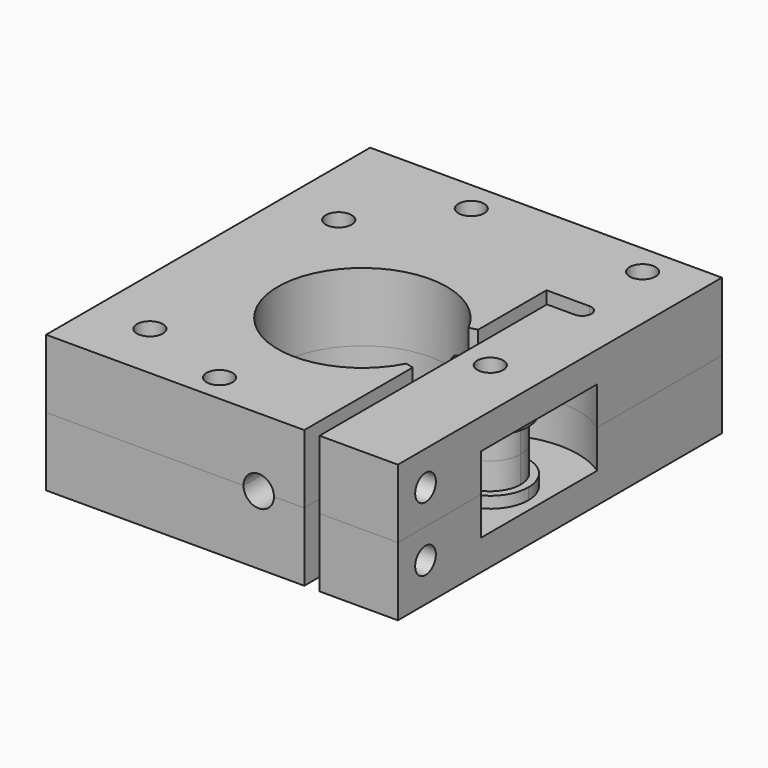
from build123d import *

# Parameters (mm, degrees)
F0_R           = 1.7
F0_R_2         = 1.35
F1_DEPTH       = 9
F2_R           = 11.1
F2_R_2         = 1.7
F3_DEPTH       = 9.001
F5_DEPTH       = 5
F6_DEPTH       = 3.5
F11_DEPTH      = 9
F13_DEPTH      = 9.001
F14_DEPTH      = 5
F15_DEPTH      = 3.5
F18_R          = 1.4
F19_DEPTH      = 20
F18_R_2        = 1.7
F20_DEPTH      = 11
F21_DEPTH      = 20
F22_DEPTH      = 11
F4_R           = 1.4
F23_DEPTH      = 9.0010001
F4_R_2         = 1.7
F24_DEPTH      = 9.0010001
F25_T1_DEPTH   = 25.9070070941
F25_2_T1_DEPTH = 25.9070070941


# Not quite as in the source:
# - a fillet or chamfer that OpenCascade refuses, or shapes differently, is made with other operations: its cross-section is extruded or revolved along the edge and cut away or added


with BuildPart() as f1:
    # F0 (on Top) → F1 (new body)
    with BuildSketch(Plane.XY):
        with BuildLine():
            Line((21.7747555523, 35.8522933333), (-24.4267012457, 35.8522933333))
            Line((-24.4267012457, 35.8522933333), (-24.4267012457, -17.3452516382))
            Line((-24.4267012457, -17.3452516382), (9.4824641046, -17.3452516382))
            Line((9.4824641046, -17.3452516382), (9.4824641046, 22.4300473309))
            Line((9.4824641046, 22.4300473309), (15.1353199035, 22.4300473309))
            ThreePointArc((15.1353199035, 22.4300473309), (16.352897448, 21.2124697864), (15.1353199035, 19.9948922419))
            Line((15.1353199035, 19.9948922419), (11.4824641046, 19.9948922419))
            Line((11.4824641046, 19.9948922419), (11.4824641046, -17.3452516382))
            Line((11.4824641046, -17.3452516382), (21.7747555523, -17.3452516382))
            Line((21.7747555523, -17.3452516382), (21.7747555523, 35.8522933333))
        make_face()
        with Locations((-4.5850900933, -13.6724999174)):
            Circle(F0_R, mode=Mode.SUBTRACT)
        with Locations((-7.8875971958, 31.7803174257)):
            Circle(F0_R, mode=Mode.SUBTRACT)
        with Locations((14.6124028042, 31.7803174257)):
            Circle(F0_R, mode=Mode.SUBTRACT)
        with Locations((-7.8875971958, 31.7803174257)):
            Circle(F0_R)
        with Locations((-7.8875971958, 31.7803174257)):
            Circle(F0_R_2, mode=Mode.SUBTRACT)
        with Locations((14.6124028042, 31.7803174257)):
            Circle(F0_R)
        with Locations((14.6124028042, 31.7803174257)):
            Circle(F0_R_2, mode=Mode.SUBTRACT)
        with Locations((-4.5850900933, -13.6724999174)):
            Circle(F0_R)
        with Locations((-4.5850900933, -13.6724999174)):
            Circle(F0_R_2, mode=Mode.SUBTRACT)
    extrude(amount=F1_DEPTH)

    # F2 (on face) → F3 (cut, through all)
    with BuildSketch(Plane.XY.offset(9)):
        with Locations((-1.4267012457, 5.8241346851)):
            Circle(F2_R)
        with Locations((-16.9267012457, 21.3241346851)):
            Circle(F2_R_2)
        with Locations((-16.9267012457, -9.6758653149)):
            Circle(F2_R_2)
    extrude(amount=-F3_DEPTH, mode=Mode.SUBTRACT)

    # F4 (on face) → F5 (cut)
    with BuildSketch(Plane.XY.offset(9)):
        with BuildLine():
            Line((11.4824641046, 8.9644222084), (11.4824641046, 16.6459370178))
            ThreePointArc((11.4824641046, 16.6459370178), (10.4596854864, 16.2215576665), (9.4824641046, 15.700777188))
            Line((9.4824641046, 15.700777188), (9.4824641046, 7.873552007))
            ThreePointArc((9.4824641046, 7.873552007), (8.4835434412, 10.8238397011), (6.7042511353, 13.380430959))
            ThreePointArc((6.7042511353, 13.380430959), (3.8732987543, 5.8241346851), (6.7042511353, -1.7321615888))
            ThreePointArc((6.7042511353, -1.7321615888), (8.4835434412, 0.8244296691), (9.4824641046, 3.7747173632))
            Line((9.4824641046, 3.7747173632), (9.4824641046, -4.0525078178))
            ThreePointArc((9.4824641046, -4.0525078178), (10.4596854864, -4.5732882963), (11.4824641046, -4.9976676476))
            Line((11.4824641046, -4.9976676476), (11.4824641046, 2.6838471618))
            ThreePointArc((11.4824641046, 2.6838471618), (10.3732987543, 5.8241346851), (11.4824641046, 8.9644222084))
        make_face()
        with BuildLine():
            Line((21.7747555523, -3.7294693921), (21.7747555523, 15.3777387623))
            ThreePointArc((21.7747555523, 15.3777387623), (16.7796726722, 17.2378156165), (11.4824641046, 16.6459370178))
            Line((11.4824641046, 16.6459370178), (11.4824641046, 8.9644222084))
            ThreePointArc((11.4824641046, 8.9644222084), (17.0385054609, 10.5386958125), (20.3732987543, 5.8241346851))
            ThreePointArc((20.3732987543, 5.8241346851), (17.0385054609, 1.1095735577), (11.4824641046, 2.6838471618))
            Line((11.4824641046, 2.6838471618), (11.4824641046, -4.9976676476))
            ThreePointArc((11.4824641046, -4.9976676476), (16.7796726722, -5.5895462463), (21.7747555523, -3.7294693921))
        make_face()
    extrude(amount=-F5_DEPTH, mode=Mode.SUBTRACT)

    # F4 (on face) → F6 (cut)
    with BuildSketch(Plane.XY.offset(9)):
        with BuildLine():
            Line((11.4824641046, 6.7522541434), (11.4824641046, 8.9644222084))
            ThreePointArc((11.4824641046, 8.9644222084), (10.3732987543, 5.8241346851), (11.4824641046, 2.6838471618))
            Line((11.4824641046, 2.6838471618), (11.4824641046, 4.8960152268))
            ThreePointArc((11.4824641046, 4.8960152268), (11.3732987543, 5.8241346851), (11.4824641046, 6.7522541434))
        make_face()
        with BuildLine():
            ThreePointArc((20.3732987543, 5.8241346851), (17.0385054609, 10.5386958125), (11.4824641046, 8.9644222084))
            Line((11.4824641046, 8.9644222084), (11.4824641046, 6.7522541434))
            ThreePointArc((11.4824641046, 6.7522541434), (15.8405574628, 9.7967496047), (19.3732987543, 5.8241346851))
            ThreePointArc((19.3732987543, 5.8241346851), (15.8405574628, 1.8515197655), (11.4824641046, 4.8960152268))
            Line((11.4824641046, 4.8960152268), (11.4824641046, 2.6838471618))
            ThreePointArc((11.4824641046, 2.6838471618), (17.0385054609, 1.1095735577), (20.3732987543, 5.8241346851))
        make_face()
    extrude(amount=-F6_DEPTH, mode=Mode.SUBTRACT)


with BuildPart() as f8:
    # F7 (on face) → F8 (revolve)
    with BuildSketch(Plane.XY.offset(9)):
        Polygon((1.5, 13.6120927054), (3.5, 13.6120927054), (3.5, 36.5408211946), (-2.6, 36.5408211946), (-2.6, 32.3408211946), (-4.7, 32.3408211946), (-4.7, 27.8408211946), (1.5, 27.8408211946), align=None)
    revolve(axis=Axis((3.5, 25.07645695, 9), (0, 1, 0)))


with BuildPart() as f8b:
    # F7 (on face) → F8, piece 2 (revolve)
    with BuildSketch(Plane.XY.offset(9)):
        Polygon((3.5, -24.8925518245), (3.5, -1.9638233352), (1.9, -1.9638233352), (1.9, -2.2529622074), (1.5, -2.2529622074), (1.5, -6.4595437571), (1.5, -11.6595437571), (1.5, -24.8925518245), align=None)
    revolve(axis=Axis((3.5, 25.07645695, 9), (0, 1, 0)))


with BuildPart() as f1_1:
    add(f1.part)

    # F9: cut F8
    add(f8.part, mode=Mode.SUBTRACT)

    # F10: cut F8b
    add(f8b.part, mode=Mode.SUBTRACT)

    # F18 (on face) → F21 (cut)
    with BuildSketch(Plane.YZ.offset(21.7747555523)):
        with Locations((-12.805685401, 5.0852382556)):
            Circle(F18_R)
    extrude(amount=-F21_DEPTH, mode=Mode.SUBTRACT)

    # F18 (on face) → F22 (cut)
    with BuildSketch(Plane.YZ.offset(21.7747555523)):
        with Locations((-12.805685401, 5.0852382556)):
            Circle(F18_R_2)
        with Locations((-12.805685401, 5.0852382556)):
            Circle(F18_R, mode=Mode.SUBTRACT)
    extrude(amount=-F22_DEPTH, mode=Mode.SUBTRACT)

    # F4 (on face) → F23 (cut, through all)
    with BuildSketch(Plane.XY.offset(9)):
        with Locations((15.3732987543, 5.8241346851)):
            Circle(F4_R)
    extrude(amount=-F23_DEPTH, mode=Mode.SUBTRACT)

    # F25: chamfer of 6 on 2 edges, made by hand

    # F25_s2 → F25_t1 (cut)
    with BuildSketch(Plane.XY.offset(-8.453503547)):
        with BuildLine():
            Line((8.1945876053, 10.8760673026), (9.7156342702, 11.2469045278))
            Line((9.7156342702, 11.2469045278), (9.8356342702, 11.2469045278))
            ThreePointArc((9.8356342702, 11.2469045278), (9.6024641046, 9.5602282674), (9.6024641046, 7.873552007))
            Line((9.6024641046, 7.873552007), (9.3645271819, 7.8513961441))
            ThreePointArc((9.3645271819, 7.8513961441), (8.9500807638, 9.4133957688), (8.0880529132, 10.8208372439))
            Line((8.0880529132, 10.8208372439), (8.1945876053, 10.8760673026))
        make_face()
        with BuildLine():
            Line((9.7156342702, 0.4013648424), (8.1945876053, 0.7722020676))
            Line((8.1945876053, 0.7722020676), (8.0880529132, 0.8274321263))
            ThreePointArc((8.0880529132, 0.8274321263), (8.9500807638, 2.2348736014), (9.3645271819, 3.7968732261))
            Line((9.3645271819, 3.7968732261), (9.6024641046, 3.7747173632))
            ThreePointArc((9.6024641046, 3.7747173632), (9.6024641046, 2.0880411028), (9.8356342702, 0.4013648424))
            Line((9.8356342702, 0.4013648424), (9.7156342702, 0.4013648424))
        make_face()
    extrude(amount=F25_T1_DEPTH, mode=Mode.SUBTRACT)


with BuildPart() as f11:
    # F0 (on Top) → F11 (new body)
    with BuildSketch(Plane.XY):
        with BuildLine():
            Line((21.7747555523, 35.8522933333), (-24.4267012457, 35.8522933333))
            Line((-24.4267012457, 35.8522933333), (-24.4267012457, -17.3452516382))
            Line((-24.4267012457, -17.3452516382), (9.4824641046, -17.3452516382))
            Line((9.4824641046, -17.3452516382), (9.4824641046, 22.4300473309))
            Line((9.4824641046, 22.4300473309), (15.1353199035, 22.4300473309))
            ThreePointArc((15.1353199035, 22.4300473309), (16.352897448, 21.2124697864), (15.1353199035, 19.9948922419))
            Line((15.1353199035, 19.9948922419), (11.4824641046, 19.9948922419))
            Line((11.4824641046, 19.9948922419), (11.4824641046, -17.3452516382))
            Line((11.4824641046, -17.3452516382), (21.7747555523, -17.3452516382))
            Line((21.7747555523, -17.3452516382), (21.7747555523, 35.8522933333))
        make_face()
        with Locations((-4.5850900933, -13.6724999174)):
            Circle(F0_R, mode=Mode.SUBTRACT)
        with Locations((-7.8875971958, 31.7803174257)):
            Circle(F0_R, mode=Mode.SUBTRACT)
        with Locations((14.6124028042, 31.7803174257)):
            Circle(F0_R, mode=Mode.SUBTRACT)
    extrude(amount=-F11_DEPTH)


with BuildPart() as f11_1:
    # F12: moved
    add(f11.part.moved(Location((0, 0, 18))))


with BuildPart() as f13_tool:
    # F2 (on face) → F13 (new body, through all)
    with BuildSketch(Plane.XY.offset(9)):
        with Locations((-1.4267012457, 5.8241346851)):
            Circle(F2_R)
        with Locations((-16.9267012457, 21.3241346851)):
            Circle(F2_R_2)
        with Locations((-16.9267012457, -9.6758653149)):
            Circle(F2_R_2)
    extrude(amount=F13_DEPTH)


with BuildPart() as f8_1:
    add(f8.part)

    # F13: cut by f13_tool
    add(f13_tool.part, mode=Mode.SUBTRACT)


with BuildPart() as f8b_1:
    add(f8b.part)

    # F13: cut by f13_tool
    add(f13_tool.part, mode=Mode.SUBTRACT)


with BuildPart() as f11_2:
    add(f11_1.part)

    # F13: cut by f13_tool
    add(f13_tool.part, mode=Mode.SUBTRACT)

    # F4 (on face) → F14 (cut)
    with BuildSketch(Plane.XY.offset(9)):
        with BuildLine():
            Line((21.7747555523, -3.7294693921), (21.7747555523, 15.3777387623))
            ThreePointArc((21.7747555523, 15.3777387623), (16.7796726722, 17.2378156165), (11.4824641046, 16.6459370178))
            Line((11.4824641046, 16.6459370178), (11.4824641046, 8.9644222084))
            ThreePointArc((11.4824641046, 8.9644222084), (17.0385054609, 10.5386958125), (20.3732987543, 5.8241346851))
            ThreePointArc((20.3732987543, 5.8241346851), (17.0385054609, 1.1095735577), (11.4824641046, 2.6838471618))
            Line((11.4824641046, 2.6838471618), (11.4824641046, -4.9976676476))
            ThreePointArc((11.4824641046, -4.9976676476), (16.7796726722, -5.5895462463), (21.7747555523, -3.7294693921))
        make_face()
    extrude(amount=F14_DEPTH, mode=Mode.SUBTRACT)

    # F4 (on face) → F15 (cut)
    with BuildSketch(Plane.XY.offset(9)):
        with BuildLine():
            Line((11.4824641046, 6.7522541434), (11.4824641046, 8.9644222084))
            ThreePointArc((11.4824641046, 8.9644222084), (10.3732987543, 5.8241346851), (11.4824641046, 2.6838471618))
            Line((11.4824641046, 2.6838471618), (11.4824641046, 4.8960152268))
            ThreePointArc((11.4824641046, 4.8960152268), (11.3732987543, 5.8241346851), (11.4824641046, 6.7522541434))
        make_face()
        with BuildLine():
            ThreePointArc((20.3732987543, 5.8241346851), (17.0385054609, 10.5386958125), (11.4824641046, 8.9644222084))
            Line((11.4824641046, 8.9644222084), (11.4824641046, 6.7522541434))
            ThreePointArc((11.4824641046, 6.7522541434), (15.8405574628, 9.7967496047), (19.3732987543, 5.8241346851))
            ThreePointArc((19.3732987543, 5.8241346851), (15.8405574628, 1.8515197655), (11.4824641046, 4.8960152268))
            Line((11.4824641046, 4.8960152268), (11.4824641046, 2.6838471618))
            ThreePointArc((11.4824641046, 2.6838471618), (17.0385054609, 1.1095735577), (20.3732987543, 5.8241346851))
        make_face()
    extrude(amount=F15_DEPTH, mode=Mode.SUBTRACT)

    # F16: cut F8
    add(f8_1.part, mode=Mode.SUBTRACT)

    # F17: cut F8b
    add(f8b_1.part, mode=Mode.SUBTRACT)

    # F18 (on face) → F19 (cut)
    with BuildSketch(Plane.YZ.offset(21.7747555523)):
        with Locations((-12.805685401, 13.5170314461)):
            Circle(F18_R)
    extrude(amount=-F19_DEPTH, mode=Mode.SUBTRACT)

    # F18 (on face) → F20 (cut)
    with BuildSketch(Plane.YZ.offset(21.7747555523)):
        with Locations((-12.805685401, 13.5170314461)):
            Circle(F18_R_2)
        with Locations((-12.805685401, 13.5170314461)):
            Circle(F18_R, mode=Mode.SUBTRACT)
    extrude(amount=-F20_DEPTH, mode=Mode.SUBTRACT)

    # F4 (on face) → F24 (cut, through all)
    with BuildSketch(Plane.XY.offset(9)):
        with Locations((15.3732987543, 5.8241346851)):
            Circle(F4_R_2)
        with Locations((15.3732987543, 5.8241346851)):
            Circle(F4_R, mode=Mode.SUBTRACT)
        with Locations((15.3732987543, 5.8241346851)):
            Circle(F4_R)
    extrude(amount=F24_DEPTH, mode=Mode.SUBTRACT)

    # F25#2: chamfer of 6 on 2 edges, made by hand

    # F25_2_s2 → F25_2_t1 (cut)
    with BuildSketch(Plane.XY.offset(0.546496453)):
        with BuildLine():
            Line((8.1945876053, 10.8760673026), (9.7156342702, 11.2469045278))
            Line((9.7156342702, 11.2469045278), (9.8356342702, 11.2469045278))
            ThreePointArc((9.8356342702, 11.2469045278), (9.6024641046, 9.5602282674), (9.6024641046, 7.873552007))
            Line((9.6024641046, 7.873552007), (9.3645271819, 7.8513961441))
            ThreePointArc((9.3645271819, 7.8513961441), (8.9500807638, 9.4133957688), (8.0880529132, 10.8208372439))
            Line((8.0880529132, 10.8208372439), (8.1945876053, 10.8760673026))
        make_face()
        with BuildLine():
            Line((9.7156342702, 0.4013648424), (8.1945876053, 0.7722020676))
            Line((8.1945876053, 0.7722020676), (8.0880529132, 0.8274321263))
            ThreePointArc((8.0880529132, 0.8274321263), (8.9500807638, 2.2348736014), (9.3645271819, 3.7968732261))
            Line((9.3645271819, 3.7968732261), (9.6024641046, 3.7747173632))
            ThreePointArc((9.6024641046, 3.7747173632), (9.6024641046, 2.0880411028), (9.8356342702, 0.4013648424))
            Line((9.8356342702, 0.4013648424), (9.7156342702, 0.4013648424))
        make_face()
    extrude(amount=F25_2_T1_DEPTH, mode=Mode.SUBTRACT)


solid = Compound([f1_1.part, f11_2.part])
